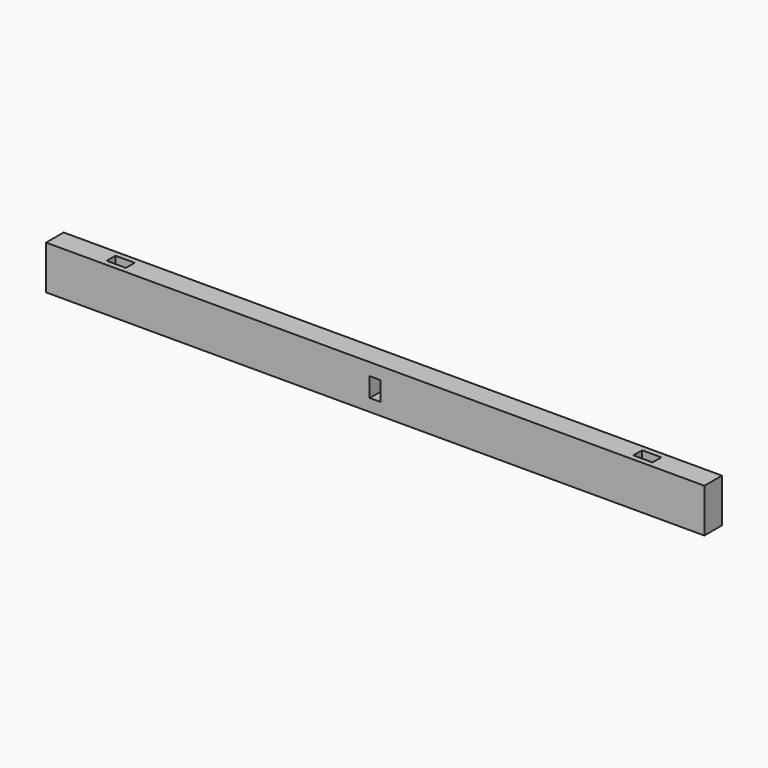
from build123d import *

# Parameters (mm, degrees)
F0_W     = 50.8
F0_H     = 101.6
F1_DEPTH = 762
F2_W     = 25.4
F2_H     = 44.45
F3_DEPTH = 50.801
F4_W     = 44.45
F4_H     = 25.4
F5_DEPTH = 101.601


# Not quite as in the source:
# - a pattern or mirror of a feature is missing from the dataset's text; its kind, count and spacing are read off the source's solid


with BuildPart() as f1:
    # F0 (on Right) → F1 (new body, symmetric)
    with BuildSketch(Plane.YZ):
        Rectangle(F0_W, F0_H)
    extrude(amount=F1_DEPTH, both=True)

    # F2 (on face) → F3 (cut, through all)
    with BuildSketch(Plane(origin=(0, 25.4, 0), x_dir=(-1, 0, 0), z_dir=(0, 1, 0))):
        Rectangle(F2_W, F2_H)
    extrude(amount=-F3_DEPTH, mode=Mode.SUBTRACT)

    # F4 (on face) → F5 (cut, through all)
    with BuildSketch(Plane.XY.offset(50.8)):
        with Locations((-609.6, 0)):
            Rectangle(F4_W, F4_H)
    f5 = extrude(amount=-F5_DEPTH, mode=Mode.SUBTRACT)

    # F5_copies: F5 across plane
    add(f5.mirror(Plane(origin=(0, 0, 0), x_dir=(0, 0, 1), z_dir=(1, 0, 0))), mode=Mode.SUBTRACT)


solid = f1.part
